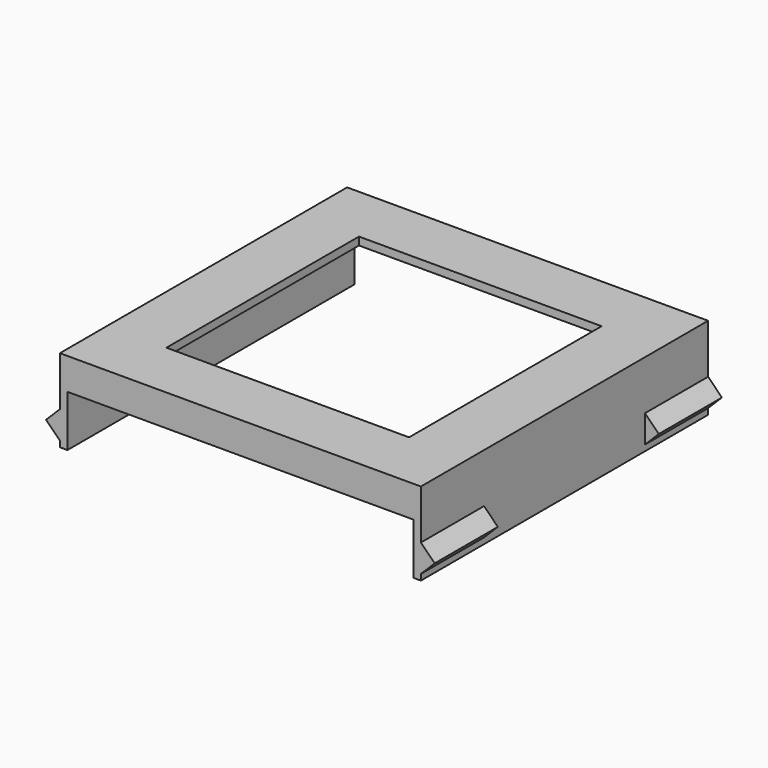
from build123d import *

# Parameters (mm, degrees)
F1_DEPTH = 45.5
F2_W     = 61.5
F2_H     = 61
F3_DEPTH = 21.001
F4_W     = 3.5
F4_H     = 51
F5_DEPTH = 21.001
F6_W     = 87.66
F6_H     = 1.44
F7_DEPTH = 6


# Not quite as in the source:
# - a pattern or mirror of a feature is missing from the dataset's text; its kind, count and spacing are read off the source's solid


with BuildPart() as f1:
    # F0 (on Front) → F1 (new body, symmetric)
    with BuildSketch(Plane.XZ):
        Polygon((45.75, 21), (-45.75, 21), (-45.75, 8.5), (-49.25, 5), (-45.75, 1.5), (-45.75, 0), (-43.83, 0), (-43.83, 19), (43.83, 19), (43.83, 0), (45.75, 0), (45.75, 1.5), (49.25, 5), (45.75, 8.5), align=None)
    extrude(amount=F1_DEPTH, both=True)

    # F2 (on face) → F3 (cut, through all)
    with BuildSketch(Plane.XY.offset(21)):
        Rectangle(F2_W, F2_H)
    extrude(amount=-F3_DEPTH, mode=Mode.SUBTRACT)

    # F4 (on face) → F5 (cut, through all)
    with BuildSketch(Plane.XY.offset(21)):
        with Locations((47.5, 0)):
            Rectangle(F4_W, F4_H)
    f5 = extrude(amount=-F5_DEPTH, mode=Mode.SUBTRACT)

    # F5_copies: F5 across plane
    add(f5.mirror(Plane(origin=(0, 0, 0), x_dir=(0, 0, -1), z_dir=(-1, 0, 0))), mode=Mode.SUBTRACT)

    # F6 (on face) → F7 (join)
    with BuildSketch(Plane(origin=(0, 0, 19), x_dir=(1, 0, 0), z_dir=(0, 0, -1))):
        with Locations((0, 44.78)):
            Rectangle(F6_W, F6_H)
    f7 = extrude(amount=F7_DEPTH)

    # F7_copies: F7 across plane
    add(f7.mirror(Plane.ZX))


solid = f1.part
